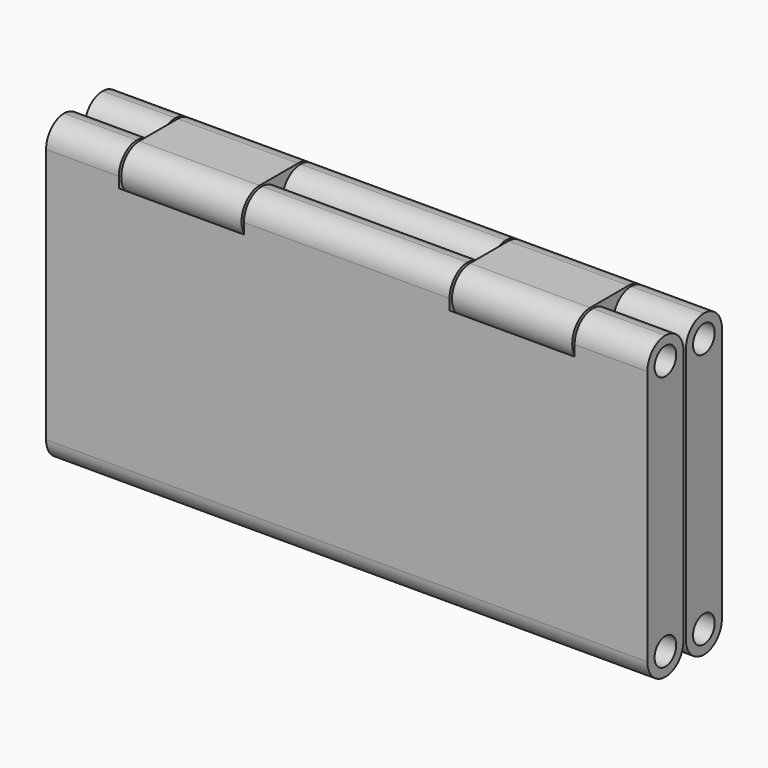
from build123d import *

# Parameters (mm, degrees)
F0_R      = 2.25
F1_DEPTH  = 50
F2_DEPTH  = 37.5
F3_DEPTH  = 17.5
F4_OFFSET = 0.4


with BuildPart() as f1:
    # F0 (on Right) → F1 (new body, symmetric)
    with BuildSketch(Plane.YZ):
        with BuildLine():
            Line((0, 46.25), (0, 3.75))
            ThreePointArc((0, 3.75), (1.0983495706, 6.4016504294), (3.75, 7.5))
            Line((3.75, 7.5), (7.5, 7.5))
            Line((7.5, 7.5), (7.5, 42.5))
            Line((7.5, 42.5), (3.75, 42.5))
            ThreePointArc((3.75, 42.5), (1.0983495706, 43.5983495706), (0, 46.25))
        make_face()
        with BuildLine():
            ThreePointArc((0, 3.75), (1.0983495706, 1.0983495706), (3.75, 0))
            ThreePointArc((3.75, 0), (6.4016504294, 1.0983495706), (7.5, 3.75))
            ThreePointArc((7.5, 3.75), (6.4016504294, 6.4016504294), (3.75, 7.5))
            ThreePointArc((3.75, 7.5), (1.0983495706, 6.4016504294), (0, 3.75))
        make_face()
        with Locations((3.75, 3.75)):
            Circle(F0_R, mode=Mode.SUBTRACT)
        with BuildLine():
            ThreePointArc((3.75, 7.5), (6.4016504294, 6.4016504294), (7.5, 3.75))
            Line((7.5, 3.75), (7.5, 7.5))
            Line((7.5, 7.5), (3.75, 7.5))
        make_face()
        with BuildLine():
            ThreePointArc((7.5, 46.25), (6.4016504294, 43.5983495706), (3.75, 42.5))
            Line((3.75, 42.5), (7.5, 42.5))
            Line((7.5, 42.5), (7.5, 46.25))
        make_face()
        with BuildLine():
            ThreePointArc((3.75, 50), (1.0983495706, 48.9016504294), (0, 46.25))
            ThreePointArc((0, 46.25), (1.0983495706, 43.5983495706), (3.75, 42.5))
            ThreePointArc((3.75, 42.5), (6.4016504294, 43.5983495706), (7.5, 46.25))
            ThreePointArc((7.5, 46.25), (6.4016504294, 48.9016504294), (3.75, 50))
        make_face()
        with Locations((3.75, 46.25)):
            Circle(F0_R, mode=Mode.SUBTRACT)
    extrude(amount=F1_DEPTH, both=True)


with BuildPart() as f1b:
    # F0 (on Right) → F1, piece 2 (new body, symmetric)
    with BuildSketch(Plane.YZ):
        with BuildLine():
            ThreePointArc((15.5, 46.25), (14.4016504294, 48.9016504294), (11.75, 50))
            ThreePointArc((11.75, 50), (9.0983495706, 48.9016504294), (8, 46.25))
            ThreePointArc((8, 46.25), (9.0983495706, 43.5983495706), (11.75, 42.5))
            ThreePointArc((11.75, 42.5), (14.4016504294, 43.5983495706), (15.5, 46.25))
        make_face()
        with Locations((11.75, 46.25)):
            Circle(F0_R, mode=Mode.SUBTRACT)
        with BuildLine():
            Line((8, 46.25), (8, 42.5))
            Line((8, 42.5), (11.75, 42.5))
            ThreePointArc((11.75, 42.5), (9.0983495706, 43.5983495706), (8, 46.25))
        make_face()
        with BuildLine():
            Line((8, 42.5), (8, 7.5))
            Line((8, 7.5), (11.75, 7.5))
            Line((11.75, 7.5), (15.5, 7.5))
            Line((15.5, 7.5), (15.5, 46.25))
            ThreePointArc((15.5, 46.25), (14.4016504294, 43.5983495706), (11.75, 42.5))
            Line((11.75, 42.5), (8, 42.5))
        make_face()
        with BuildLine():
            ThreePointArc((11.75, 7.5), (14.4016504294, 6.4016504294), (15.5, 3.75))
            Line((15.5, 3.75), (15.5, 7.5))
            Line((15.5, 7.5), (11.75, 7.5))
        make_face()
        with BuildLine():
            Line((8, 7.5), (8, 3.75))
            ThreePointArc((8, 3.75), (9.0983495706, 6.4016504294), (11.75, 7.5))
            Line((11.75, 7.5), (8, 7.5))
        make_face()
        with BuildLine():
            ThreePointArc((8, 3.75), (9.0983495706, 1.0983495706), (11.75, 0))
            ThreePointArc((11.75, 0), (14.4016504294, 1.0983495706), (15.5, 3.75))
            ThreePointArc((15.5, 3.75), (14.4016504294, 6.4016504294), (11.75, 7.5))
            ThreePointArc((11.75, 7.5), (9.0983495706, 6.4016504294), (8, 3.75))
        make_face()
        with Locations((11.75, 3.75)):
            Circle(F0_R, mode=Mode.SUBTRACT)
        with BuildLine():
            Line((8, 42.5), (8, 7.5))
            Line((8, 7.5), (11.75, 7.5))
            Line((11.75, 7.5), (15.5, 7.5))
            Line((15.5, 7.5), (15.5, 46.25))
            ThreePointArc((15.5, 46.25), (14.4016504294, 43.5983495706), (11.75, 42.5))
            Line((11.75, 42.5), (8, 42.5))
        make_face()
    extrude(amount=F1_DEPTH, both=True)


with BuildPart() as f2:
    # F0 (on Right) → F2 (new body, symmetric)
    with BuildSketch(Plane.YZ):
        with BuildLine():
            ThreePointArc((3.75, 50), (1.0983495706, 48.9016504294), (0, 46.25))
            ThreePointArc((0, 46.25), (1.0983495706, 43.5983495706), (3.75, 42.5))
            ThreePointArc((3.75, 42.5), (6.4016504294, 43.5983495706), (7.5, 46.25))
            ThreePointArc((7.5, 46.25), (6.4016504294, 48.9016504294), (3.75, 50))
        make_face()
        with Locations((3.75, 46.25)):
            Circle(F0_R, mode=Mode.SUBTRACT)
        with BuildLine():
            ThreePointArc((7.5, 46.25), (6.4016504294, 43.5983495706), (3.75, 42.5))
            Line((3.75, 42.5), (7.5, 42.5))
            Line((7.5, 42.5), (7.5, 46.25))
        make_face()
        with BuildLine():
            Line((7.5, 46.25), (7.5, 42.5))
            Line((7.5, 42.5), (8, 42.5))
            Line((8, 42.5), (8, 46.25))
            ThreePointArc((8, 46.25), (9.0983495706, 48.9016504294), (11.75, 50))
            Line((11.75, 50), (7.5, 50))
            Line((7.5, 50), (7.5, 46.25))
        make_face()
        with BuildLine():
            Line((8, 46.25), (8, 42.5))
            Line((8, 42.5), (11.75, 42.5))
            ThreePointArc((11.75, 42.5), (9.0983495706, 43.5983495706), (8, 46.25))
        make_face()
        with BuildLine():
            Line((7.5, 50), (3.75, 50))
            ThreePointArc((3.75, 50), (6.4016504294, 48.9016504294), (7.5, 46.25))
            Line((7.5, 46.25), (7.5, 50))
        make_face()
        with BuildLine():
            ThreePointArc((15.5, 46.25), (14.4016504294, 48.9016504294), (11.75, 50))
            ThreePointArc((11.75, 50), (9.0983495706, 48.9016504294), (8, 46.25))
            ThreePointArc((8, 46.25), (9.0983495706, 43.5983495706), (11.75, 42.5))
            ThreePointArc((11.75, 42.5), (14.4016504294, 43.5983495706), (15.5, 46.25))
        make_face()
        with Locations((11.75, 46.25)):
            Circle(F0_R, mode=Mode.SUBTRACT)
    extrude(amount=F2_DEPTH, both=True)

    # F0 (on Right) → F3 (cut, symmetric)
    with BuildSketch(Plane.YZ):
        with BuildLine():
            ThreePointArc((3.75, 50), (1.0983495706, 48.9016504294), (0, 46.25))
            ThreePointArc((0, 46.25), (1.0983495706, 43.5983495706), (3.75, 42.5))
            ThreePointArc((3.75, 42.5), (6.4016504294, 43.5983495706), (7.5, 46.25))
            ThreePointArc((7.5, 46.25), (6.4016504294, 48.9016504294), (3.75, 50))
        make_face()
        with Locations((3.75, 46.25)):
            Circle(F0_R, mode=Mode.SUBTRACT)
        with BuildLine():
            Line((7.5, 50), (3.75, 50))
            ThreePointArc((3.75, 50), (6.4016504294, 48.9016504294), (7.5, 46.25))
            Line((7.5, 46.25), (7.5, 50))
        make_face()
        with BuildLine():
            Line((7.5, 46.25), (7.5, 42.5))
            Line((7.5, 42.5), (8, 42.5))
            Line((8, 42.5), (8, 46.25))
            ThreePointArc((8, 46.25), (9.0983495706, 48.9016504294), (11.75, 50))
            Line((11.75, 50), (7.5, 50))
            Line((7.5, 50), (7.5, 46.25))
        make_face()
        with BuildLine():
            ThreePointArc((15.5, 46.25), (14.4016504294, 48.9016504294), (11.75, 50))
            ThreePointArc((11.75, 50), (9.0983495706, 48.9016504294), (8, 46.25))
            ThreePointArc((8, 46.25), (9.0983495706, 43.5983495706), (11.75, 42.5))
            ThreePointArc((11.75, 42.5), (14.4016504294, 43.5983495706), (15.5, 46.25))
        make_face()
        with Locations((11.75, 46.25)):
            Circle(F0_R, mode=Mode.SUBTRACT)
        with BuildLine():
            Line((8, 46.25), (8, 42.5))
            Line((8, 42.5), (11.75, 42.5))
            ThreePointArc((11.75, 42.5), (9.0983495706, 43.5983495706), (8, 46.25))
        make_face()
        with BuildLine():
            ThreePointArc((7.5, 46.25), (6.4016504294, 43.5983495706), (3.75, 42.5))
            Line((3.75, 42.5), (7.5, 42.5))
            Line((7.5, 42.5), (7.5, 46.25))
        make_face()
    extrude(amount=F3_DEPTH, both=True, mode=Mode.SUBTRACT)


with BuildPart() as f1_1:
    add(f1.part)

    # F4: cut F2, made larger all round first
    f4_tool = offset(f2.part, amount=F4_OFFSET, kind=Kind.INTERSECTION, mode=Mode.PRIVATE)
    add(f4_tool, mode=Mode.SUBTRACT)


with BuildPart() as f1b_1:
    add(f1b.part)

    # F4: cut F2, made larger all round first
    f4_tool = offset(f2.part, amount=F4_OFFSET, kind=Kind.INTERSECTION, mode=Mode.PRIVATE)
    add(f4_tool, mode=Mode.SUBTRACT)


solid = Compound([f2.part, f1_1.part, f1b_1.part])
